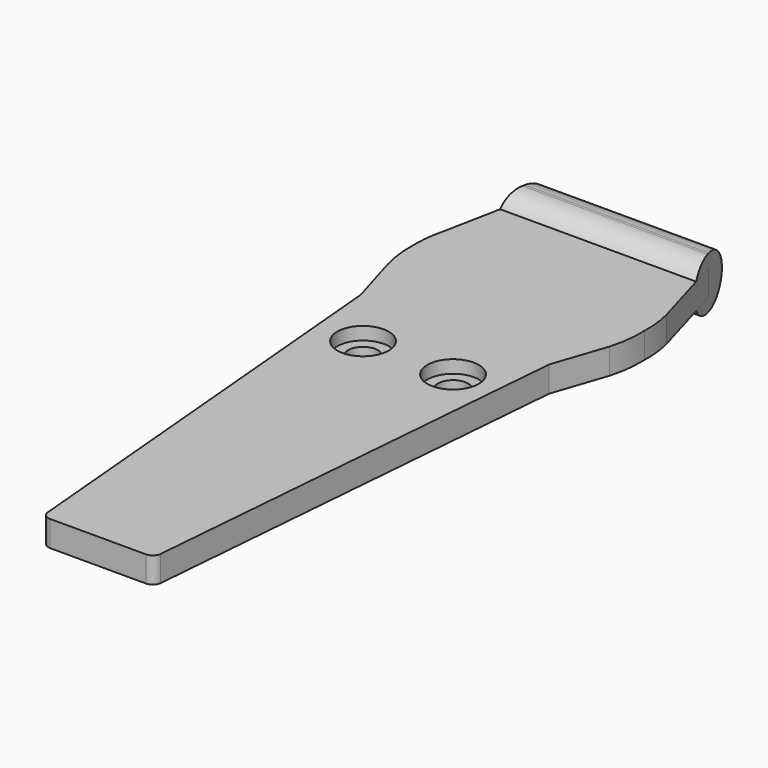
from build123d import *

# Parameters (mm, degrees)
F0_R          = 1.75
F1_DEPTH      = 3
F3_DEPTH      = 1.5
F3_DEPTH_BACK = 4.5
F4_T1_DEPTH   = 35.8553046099
F4_T3_DEPTH   = 35
F5_R          = 3
F6_DEPTH      = 1.5


# Not quite as in the source:
# - a fillet or chamfer that OpenCascade refuses, or shapes differently, is made with other operations: its cross-section is extruded or revolved along the edge and cut away or added
# - a feature names something its author has since deleted; it is built from what else it names


with BuildPart() as f1:
    # F0 (on Top) → F1 (new body)
    with BuildSketch(Plane.XY):
        with BuildLine():
            Line((-5.5846913819, -42.1934081889), (5.5801667099, -42.1934081889))
            ThreePointArc((5.5801667099, -42.1934081889), (6.2571567858, -41.9294003336), (6.5766854657, -41.2767770629))
            Line((6.5766854657, -41.2767770629), (10.8664863973, 9.9997591089))
            Line((10.8664863973, 9.9997591089), (12.9481358013, 16.1793168214))
            ThreePointArc((12.9481358013, 16.1793168214), (13.3997566467, 18.3576501573), (13.4874998392, 20.5805758517))
            Line((13.4874998392, 20.5805758517), (13.4943094486, 20.6080656878))
            ThreePointArc((13.4943094486, 20.6080656878), (13.4214184301, 22.4544852439), (13.0970679667, 24.2736540252))
            Line((13.0970679667, 24.2736540252), (10.3058793621, 33.9058264779))
            Line((10.3058793621, 33.9058264779), (9.4093267365, 36.9997591089))
            Line((9.4093267365, 36.9997591089), (4.9829727946, 36.9997591089))
            Line((4.9829727946, 36.9997591089), (-5.25, 36.9997591089))
            Line((-5.25, 36.9997591089), (-10.5906732635, 36.9997591089))
            Line((-10.5906732635, 36.9997591089), (-10.7942270682, 35.9658364889))
            Line((-10.7942270682, 35.9658364889), (-13.0926909538, 24.2911158576))
            Line((-13.0926909538, 24.2911158576), (-13.3631447598, 22.9173841889))
            ThreePointArc((-13.3631447598, 22.9173841889), (-13.4782769531, 21.765539271), (-13.4943094486, 20.6080656878))
            Line((-13.4943094486, 20.6080656878), (-13.4876078419, 20.5780624058))
            ThreePointArc((-13.4876078419, 20.5780624058), (-13.3996035826, 18.3564016222), (-12.9481358013, 16.1793168214))
            Line((-12.9481358013, 16.1793168214), (-11.1248120452, 9.9997591089))
            Line((-11.1248120452, 9.9997591089), (-6.5807885254, -41.281671889))
            ThreePointArc((-6.5807885254, -41.281671889), (-6.259871469, -41.9310611222), (-5.5846913819, -42.1934081889))
        make_face()
        with Locations((-5.25, 2.9997591089)):
            Circle(F0_R, mode=Mode.SUBTRACT)
        with Locations((5.25, 2.9997591089)):
            Circle(F0_R, mode=Mode.SUBTRACT)
        with BuildLine():
            ThreePointArc((-13.0926909538, 24.2911158576), (-13.2457387677, 23.6077585201), (-13.3631447598, 22.9173841889))
            Line((-13.3631447598, 22.9173841889), (-13.0926909538, 24.2911158576))
        make_face()
    extrude(amount=F1_DEPTH)

    # F2 (on face) → F3 (join, two sides)
    with BuildSketch(Plane.XY.offset(3)) as f3_sk:
        Polygon((9.4093267365, 36.9997591089), (-10.5906732635, 36.9997591089), (-11.7496770502, 31.1127641011), (11.1152465029, 31.1127641011), align=None)
    extrude(amount=F3_DEPTH)
    extrude(f3_sk.sketch, amount=-F3_DEPTH_BACK)

    # F4: fillet of radius 3 on 4 edges, made by hand

    # F4_s2 → F4_t1 (cut)
    with BuildSketch(Plane.YZ.offset(-18.2448675786)):
        with BuildLine():
            ThreePointArc((33.7108403124, 4.5), (32.2108403124, 4.0980762114), (31.1127641011, 3))
            Line((31.1127641011, 3), (31.1127641011, 4.5))
            Line((31.1127641011, 4.5), (33.7108403124, 4.5))
        make_face()
        with BuildLine():
            ThreePointArc((31.1127641011, 0), (32.2108403124, -1.0980762114), (33.7108403124, -1.5))
            Line((33.7108403124, -1.5), (31.1127641011, -1.5))
            Line((31.1127641011, -1.5), (31.1127641011, 0))
        make_face()
    extrude(amount=F4_T1_DEPTH, mode=Mode.SUBTRACT)

    # F4_s4 → F4_t3 (cut)
    with BuildSketch(Plane.YZ.offset(-18.0906732635)):
        with BuildLine():
            ThreePointArc((36.9997591089, 1.5), (36.1210794525, 3.6213203436), (33.9997591089, 4.5))
            Line((33.9997591089, 4.5), (36.9997591089, 4.5))
            Line((36.9997591089, 4.5), (36.9997591089, 1.5))
        make_face()
        with BuildLine():
            ThreePointArc((33.9997591089, -1.5), (36.1210794525, -0.6213203436), (36.9997591089, 1.5))
            Line((36.9997591089, 1.5), (36.9997591089, -1.5))
            Line((36.9997591089, -1.5), (33.9997591089, -1.5))
        make_face()
    extrude(amount=F4_T3_DEPTH, mode=Mode.SUBTRACT)

    # F5 (on face) → F6 (cut)
    with BuildSketch(Plane.XY.offset(3)):
        with Locations((-5.25, 2.9997591089)):
            Circle(F5_R)
        with Locations((5.25, 2.9997591089)):
            Circle(F5_R)
    extrude(amount=-F6_DEPTH, mode=Mode.SUBTRACT)


solid = f1.part
